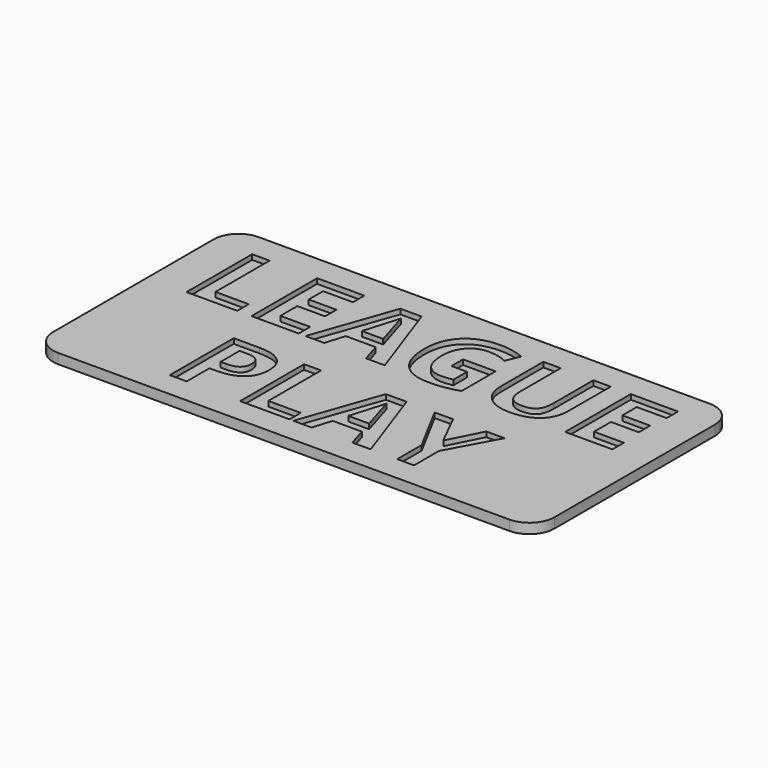
from build123d import *

# Parameters (mm, degrees)
F1_DEPTH       = 2
F2_TEXT_SIZE   = 22.9154965685
F2_TEXT_SIZE_2 = 22.3426122425
F3_DEPTH       = 1


# Not quite as in the source:
# - Text() gives the source's letters only with a copy of the font that has no kerning and outlines rounded to 1/6400 em; it was checked with that copy


with BuildPart() as f1:
    # F0 (on Top) → F1 (new body)
    with BuildSketch(Plane.XY):
        with BuildLine():
            Line((-45, -25), (45, -25))
            ThreePointArc((45, -25), (48.5355339059, -23.5355339059), (50, -20))
            Line((50, -20), (50, 20))
            ThreePointArc((50, 20), (48.5355339059, 23.5355339059), (45, 25))
            Line((45, 25), (-45, 25))
            ThreePointArc((-45, 25), (-48.5355339059, 23.5355339059), (-50, 20))
            Line((-50, 20), (-50, -20))
            ThreePointArc((-50, -20), (-48.5355339059, -23.5355339059), (-45, -25))
        make_face()
    extrude(amount=F1_DEPTH)

    # F2 (on face) → F3 (cut)
    with BuildSketch(Plane.XY.offset(2)):
        with Locations((-44.2358597431, 3.5008424707)):
            Text('LEAGUE', F2_TEXT_SIZE, font='Open Sans', font_style=FontStyle.BOLD, text_align=(TextAlign.LEFT, TextAlign.BOTTOM))
        with Locations((-28.7312029306, -20)):
            Text('PLAY', F2_TEXT_SIZE_2, font='Open Sans', font_style=FontStyle.BOLD, text_align=(TextAlign.LEFT, TextAlign.BOTTOM))
    extrude(amount=-F3_DEPTH, mode=Mode.SUBTRACT)


solid = f1.part
